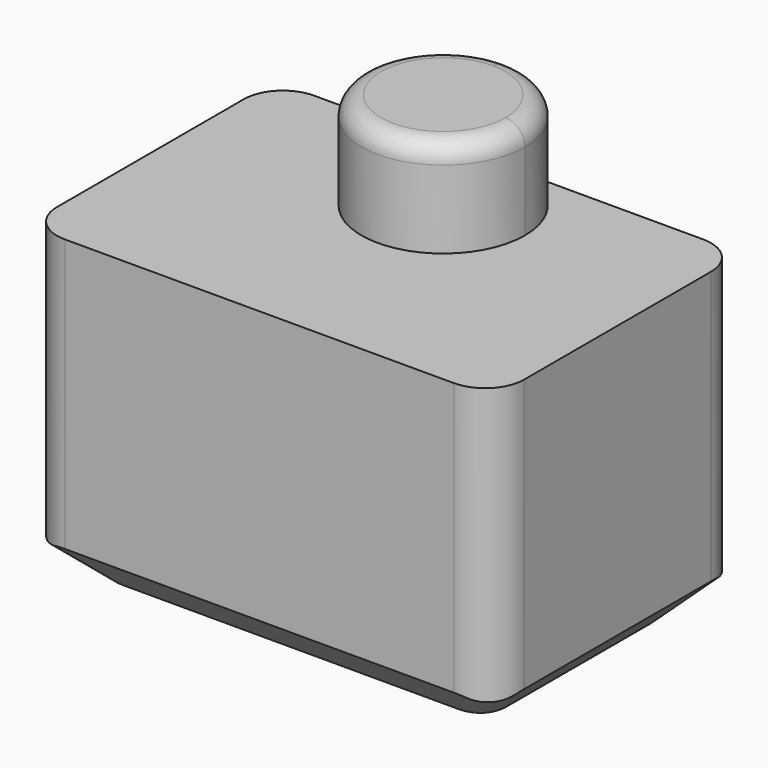
from build123d import *

# Parameters (mm, degrees)
F1_DEPTH = 8
F2_DEPTH = 2.5
F3_R     = 0.5
F4_SIZE  = 1
F5_F1_R  = 1
F5_F2_R  = 1
F5_F3_R  = 1
F5_F4_R  = 1
F5_F5_R  = 1
F5_F6_R  = 1
F5_F7_R  = 1
F5_F8_R  = 1


with BuildPart() as f1:
    # F0 (on Top) → F1 (new body)
    with BuildSketch(Plane.XY):
        Polygon((-6, -4), (6, -4), (6, 4), (0, 4), (-6, 4), align=None)
        with BuildLine():
            ThreePointArc((2.1, 1.9), (-1.4849242405, 0.4150757595), (0, 4))
            ThreePointArc((0, 4), (1.4849242405, 3.3849242405), (2.1, 1.9))
        make_face(mode=Mode.SUBTRACT)
        with BuildLine():
            ThreePointArc((2.1, 1.9), (1.4849242405, 3.3849242405), (0, 4))
            ThreePointArc((0, 4), (-1.4849242405, 0.4150757595), (2.1, 1.9))
        make_face()
    extrude(amount=-F1_DEPTH)

    # F0 (on Top) → F2 (join)
    with BuildSketch(Plane.XY):
        with BuildLine():
            ThreePointArc((2.1, 1.9), (1.4849242405, 3.3849242405), (0, 4))
            ThreePointArc((0, 4), (-1.4849242405, 0.4150757595), (2.1, 1.9))
        make_face()
    extrude(amount=F2_DEPTH)

    # F3
    f3_edges = [f1.edges().sort_by_distance(p)[0] for p in [
        (-2.1, 1.9, 2.5),
    ]]
    fillet(f3_edges, radius=F3_R)

    # F4
    f4_edges = [f1.edges().sort_by_distance(p)[0] for p in [
        (-6, 0, -8),
        (0, -4, -8),
        (0, 4, -8),
        (6, 0, -8),
    ]]
    chamfer(f4_edges, length=F4_SIZE)

    # F5: fillet of radius 1 on 8 edges, made by hand

    # F5_f1
    f5_f1_edges = [f1.edges().sort_by_distance(p)[0] for p in [
        (6, 4, -3.5),
    ]]
    fillet(f5_f1_edges, radius=F5_F1_R)

    # F5_f2
    f5_f2_edges = [f1.edges().sort_by_distance(p)[0] for p in [
        (-6, 4, -3.5),
    ]]
    fillet(f5_f2_edges, radius=F5_F2_R)

    # F5_f3
    f5_f3_edges = [f1.edges().sort_by_distance(p)[0] for p in [
        (6, -4, -3.5),
    ]]
    fillet(f5_f3_edges, radius=F5_F3_R)

    # F5_f4
    f5_f4_edges = [f1.edges().sort_by_distance(p)[0] for p in [
        (5.3535533906, 3.3535533906, -7.6464466094),
    ]]
    fillet(f5_f4_edges, radius=F5_F4_R)

    # F5_f5
    f5_f5_edges = [f1.edges().sort_by_distance(p)[0] for p in [
        (-5.3535533906, 3.3535533906, -7.6464466094),
    ]]
    fillet(f5_f5_edges, radius=F5_F5_R)

    # F5_f6
    f5_f6_edges = [f1.edges().sort_by_distance(p)[0] for p in [
        (-6, -4, -3.5),
    ]]
    fillet(f5_f6_edges, radius=F5_F6_R)

    # F5_f7
    f5_f7_edges = [f1.edges().sort_by_distance(p)[0] for p in [
        (5.3535533906, -3.3535533906, -7.6464466094),
    ]]
    fillet(f5_f7_edges, radius=F5_F7_R)

    # F5_f8
    f5_f8_edges = [f1.edges().sort_by_distance(p)[0] for p in [
        (-5.3535533906, -3.3535533906, -7.6464466094),
    ]]
    fillet(f5_f8_edges, radius=F5_F8_R)


solid = f1.part
